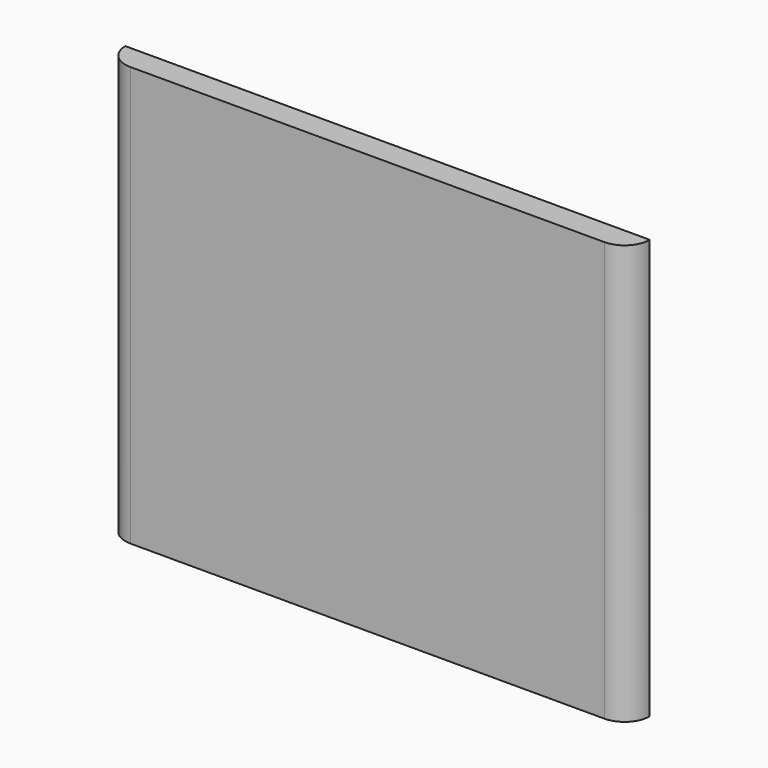
from build123d import *

# Parameters (mm, degrees)
F0_W     = 396.875
F0_H     = 317.5
F1_DEPTH = 19.05
F2_R     = 19.04999


# Not quite as in the source:
# - a fillet or chamfer is up to 0.001 mm smaller than in the source, because OpenCascade refuses the exact size


with BuildPart() as f1:
    # F0 (on Front) → F1 (new body)
    with BuildSketch(Plane.XZ):
        Rectangle(F0_W, F0_H)
    extrude(amount=F1_DEPTH)

    # F2 (radius 19.05 in the source; OpenCascade refuses exactly that, so slightly less here)
    f2_edges = [f1.edges().sort_by_distance(p)[0] for p in [
        (-198.4375, -19.05, 0),
        (198.4375, -19.05, 0),
    ]]
    fillet(f2_edges, radius=F2_R)


solid = f1.part
